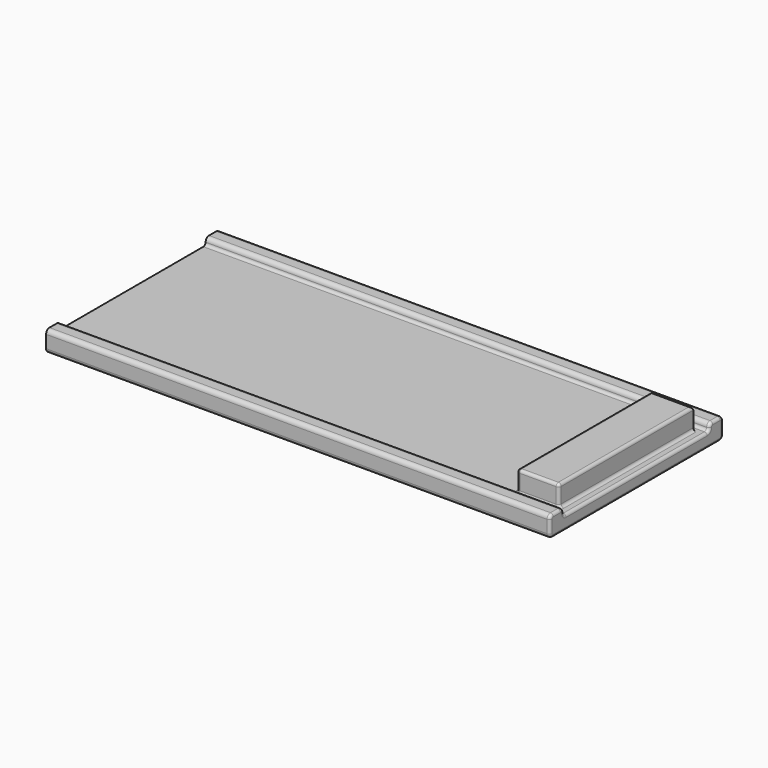
from build123d import *

# Parameters (mm, degrees)
F0_W     = 914.4
F0_H     = 393.7
F1_DEPTH = 25.4
F2_W     = 914.4
F2_H     = 31.75
F3_DEPTH = 12.7
F4_W     = 76.2
F4_H     = 304.8
F5_DEPTH = 38.1
F6_R     = 7.62
F7_R     = 5.07999


# Not quite as in the source:
# - a fillet or chamfer is up to 0.001 mm smaller than in the source, because OpenCascade refuses the exact size


with BuildPart() as f1:
    # F0 (on Top) → F1 (new body)
    with BuildSketch(Plane.XY):
        with Locations((457.2, 196.85)):
            Rectangle(F0_W, F0_H)
    extrude(amount=F1_DEPTH)

    # F2 (on face) → F3 (join)
    with BuildSketch(Plane.XY.offset(25.4)):
        with Locations((457.2, 377.825)):
            Rectangle(F2_W, F2_H)
        with Locations((457.2, 15.875)):
            Rectangle(F2_W, F2_H)
    extrude(amount=F3_DEPTH)

    # F4 (on face) → F5 (join)
    with BuildSketch(Plane.XY.offset(25.4)):
        with Locations((857.25, 196.85)):
            Rectangle(F4_W, F4_H)
    extrude(amount=F5_DEPTH)

    # F6
    f6_edges = [f1.edges().sort_by_distance(p)[0] for p in [
        (457.2, 393.7, 38.1),
        (457.2, 361.95, 38.1),
        (457.2, 31.75, 38.1),
        (457.2, 0, 38.1),
        (457.2, 393.7, 0),
        (457.2, 0, 0),
    ]]
    fillet(f6_edges, radius=F6_R)

    # F7 (radius 5.08 in the source; OpenCascade refuses exactly that, so slightly less here)
    f7_edges = [f1.edges().sort_by_distance(p)[0] for p in [
        (895.35, 196.85, 63.5),
        (857.25, 349.25, 63.5),
        (819.15, 196.85, 63.5),
        (857.25, 44.45, 63.5),
        (819.15, 44.45, 44.45),
        (895.35, 44.45, 44.45),
        (857.25, 44.45, 25.4),
        (457.2, 31.75, 25.4),
        (457.2, 361.95, 25.4),
        (914.4, 196.85, 25.4),
        (914.4, 393.7, 19.05),
        (914.4, 391.468154, 35.868154),
        (914.4, 391.468154, 2.231846),
        (914.4, 377.825, 38.1),
        (914.4, 196.85, 0),
        (914.4, 364.181846, 35.868154),
        (914.4, 2.231846, 2.231846),
        (914.4, 0, 19.05),
        (895.35, 196.85, 25.4),
        (819.15, 196.85, 25.4),
        (914.4, 2.231846, 35.868154),
        (914.4, 15.875, 38.1),
        (914.4, 29.518154, 35.868154),
    ]]
    fillet(f7_edges, radius=F7_R)


solid = f1.part
